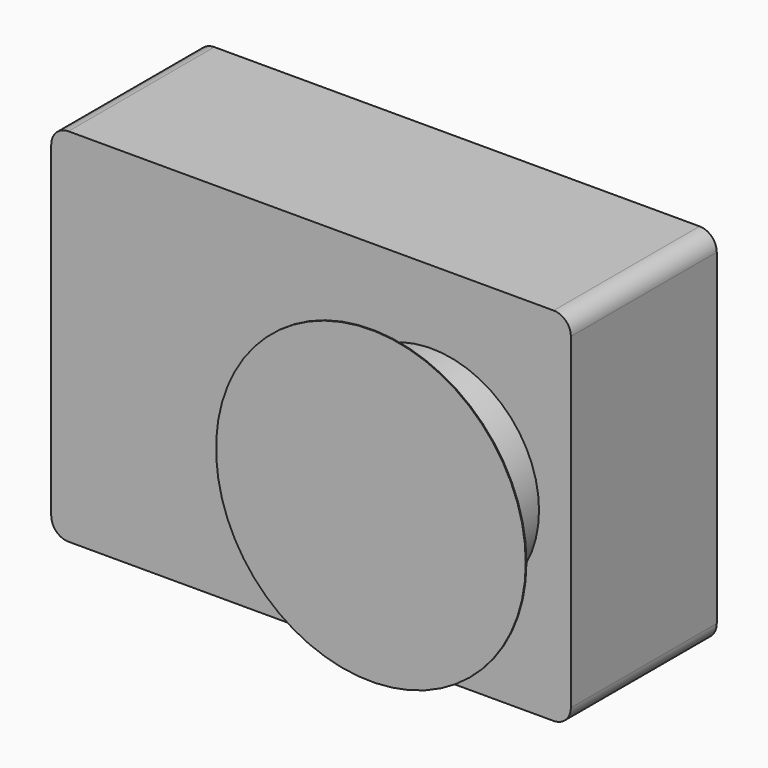
from build123d import *

# Parameters (mm, degrees)
F0_R      = 12.5
F1_DEPTH  = 30
F2_DEPTH  = 21.2
F3_R      = 2
F4_R      = 2
F5_R      = 2
F6_R      = 2
F7_R      = 13.25
F7_R_2    = 12.5
F8_DEPTH  = 3.5
F7_R_3    = 18
F7_R_4    = 17.5
F10_DEPTH = 0.1


# Not quite as in the source:
# - the program builds the solid bodies; features that only make, move or delete a surface that nothing else refers to are left out


with BuildPart() as f1:
    # F0 (on Front) → F1 (new body)
    with BuildSketch(Plane.XZ):
        with Locations((14, 0)):
            Circle(F0_R)
    extrude(amount=F1_DEPTH)

    # F0 (on Front) → F2 (join)
    with BuildSketch(Plane.XZ):
        Polygon((30.2, -21), (30.2, 0), (30.2, 21), (-30.2, 21), (-30.2, -21), align=None)
        with Locations((14, 0)):
            Circle(F0_R, mode=Mode.SUBTRACT)
    extrude(amount=F2_DEPTH)

    # F3
    f3_edges = [f1.edges().sort_by_distance(p)[0] for p in [
        (-30.2, -10.6, 21),
    ]]
    fillet(f3_edges, radius=F3_R)

    # F4
    f4_edges = [f1.edges().sort_by_distance(p)[0] for p in [
        (30.2, -10.6, 21),
    ]]
    fillet(f4_edges, radius=F4_R)

    # F5
    f5_edges = [f1.edges().sort_by_distance(p)[0] for p in [
        (-30.2, -10.6, -21),
    ]]
    fillet(f5_edges, radius=F5_R)

    # F6
    f6_edges = [f1.edges().sort_by_distance(p)[0] for p in [
        (30.2, -10.6, -21),
    ]]
    fillet(f6_edges, radius=F6_R)

    # F7 (on face) → F8 (join)
    with BuildSketch(Plane.XZ.offset(30)):
        with Locations((14, 0)):
            Circle(F7_R)
        with Locations((14, 0)):
            Circle(F7_R_2, mode=Mode.SUBTRACT)
    extrude(amount=-F8_DEPTH)

    # F7 (on face) → F10 (join)
    with BuildSketch(Plane.XZ.offset(30)):
        with Locations((14, 0)):
            Circle(F7_R_3)
        with Locations((14, 0)):
            Circle(F7_R_4, mode=Mode.SUBTRACT)
        with Locations((14, 0)):
            Circle(F7_R_4)
        with Locations((14, 0)):
            Circle(F7_R, mode=Mode.SUBTRACT)
    extrude(amount=-F10_DEPTH)


solid = f1.part
